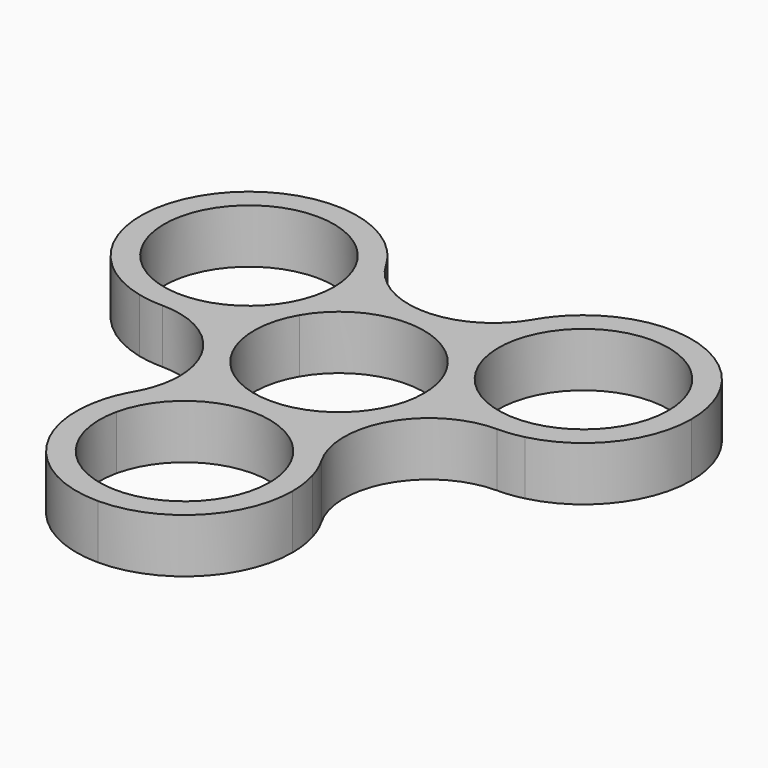
from build123d import *

# Parameters (mm, degrees)
F1_DEPTH = 7


# Not quite as in the source:
# - a feature names something its author has since deleted; it is built from what else it names


with BuildPart() as f1:
    # F0 (on Top) → F1 (new body)
    with BuildSketch(Plane.XY):
        with BuildLine():
            ThreePointArc((9.5262796516, 5.4999996362), (10.6251841435, 2.8470092933), (11, 0))
            ThreePointArc((11, 0), (7.7781745931, -7.7781745931), (0, -11))
            ThreePointArc((0, -11), (6.9999999972, -12.8756443454), (12.1243556497, -17.9999999943))
            ThreePointArc((12.1243556497, -17.9999999943), (12.1243556546, -6.9999999972), (21.6506350946, -1.5))
            ThreePointArc((21.6506350946, -1.5), (14.6506352765, 0.375644242), (9.5262796516, 5.4999996362))
        make_face()
        with BuildLine():
            ThreePointArc((-9.5262796375, 5.4999996607), (1.41e-08, 11), (9.5262796516, 5.4999996362))
            ThreePointArc((9.5262796516, 5.4999996362), (7.6506350946, 12.4999999615), (9.5262796131, 19.500000297))
            ThreePointArc((9.5262796131, 19.500000297), (-4.54e-08, 14), (-9.5262796585, 19.5000003756))
            ThreePointArc((-9.5262796585, 19.5000003756), (-8.1276735827, 16.1234668409), (-7.6506350946, 12.5))
            ThreePointArc((-7.6506350946, 12.5), (-8.1276735773, 8.8765331793), (-9.5262796375, 5.4999996607))
        make_face()
        with BuildLine():
            ThreePointArc((9.5262796131, 19.500000297), (7.6506350946, 12.4999999615), (9.5262796516, 5.4999996362))
            ThreePointArc((9.5262796516, 5.4999996362), (14.6506352765, 0.375644242), (21.6506350946, -1.5))
            ThreePointArc((21.6506350946, -1.5), (23.3252484864, -1.3994845224), (24.9758155118, -1.0993814269))
            ThreePointArc((24.9758155118, -1.0993814269), (24.9939531467, -0.5498237016), (25, 0))
            ThreePointArc((25, 0), (24.9800177424, 0.9993565887), (24.9201029127, 1.9971156254))
            ThreePointArc((24.9201029127, 1.9971156254), (12.124355653, 7), (14.1896043222, 20.5828843746))
            ThreePointArc((14.1896043222, 20.5828843746), (12.8874554167, 21.4222662872), (11.5358155118, 22.1793814269))
            ThreePointArc((11.5358155118, 22.1793814269), (10.4506351975, 20.9000001372), (9.5262796131, 19.500000297))
        make_face()
        with BuildLine():
            ThreePointArc((-12.1243556177, -17.999999939), (-6.9999999695, -12.8756443294), (0, -11))
            ThreePointArc((0, -11), (-9.5262793437, -5.5000001697), (-9.5262796375, 5.4999996607))
            ThreePointArc((-9.5262796375, 5.4999996607), (-14.6506352643, 0.3756442491), (-21.6506350946, -1.5))
            ThreePointArc((-21.6506350946, -1.5), (-13.8724605016, -4.7218254069), (-10.6506350946, -12.5))
            ThreePointArc((-10.6506350946, -12.5), (-11.0254509963, -15.3470094621), (-12.1243556177, -17.999999939))
        make_face()
        with BuildLine():
            ThreePointArc((12.1243556497, -17.9999999943), (6.9999999972, -12.8756443454), (0, -11))
            ThreePointArc((0, -11), (-6.9999999695, -12.8756443294), (-12.1243556177, -17.999999939))
            ThreePointArc((-12.1243556177, -17.999999939), (-12.8746133779, -19.5005154452), (-13.44, -21.08))
            ThreePointArc((-13.44, -21.08), (-12.108499103, -21.8719969247), (-10.7304985905, -22.58))
            ThreePointArc((-10.7304985905, -22.58), (0, -14), (10.7304985905, -22.58))
            ThreePointArc((10.7304985905, -22.58), (12.108499103, -21.8719969247), (13.44, -21.08))
            ThreePointArc((13.44, -21.08), (12.8746133905, -19.5005154746), (12.1243556497, -17.9999999943))
        make_face()
        with BuildLine():
            ThreePointArc((-21.6506350946, -1.5), (-14.6506352643, 0.3756442491), (-9.5262796375, 5.4999996607))
            ThreePointArc((-9.5262796375, 5.4999996607), (-8.1276735773, 8.8765331793), (-7.6506350946, 12.5))
            ThreePointArc((-7.6506350946, 12.5), (-8.1276735827, 16.1234668409), (-9.5262796585, 19.5000003756))
            ThreePointArc((-9.5262796585, 19.5000003756), (-10.4506352247, 20.9000001735), (-11.5358155118, 22.1793814269))
            ThreePointArc((-11.5358155118, 22.1793814269), (-12.8874554167, 21.4222662872), (-14.1896043222, 20.5828843746))
            ThreePointArc((-14.1896043222, 20.5828843746), (-11.5741441752, 16.9118398375), (-10.6506350946, 12.5))
            ThreePointArc((-10.6506350946, 12.5), (-15.1300578962, 3.6409891636), (-24.9201029127, 1.9971156254))
            ThreePointArc((-24.9201029127, 1.9971156254), (-24.9959545198, 0.4497306374), (-24.9758155118, -1.0993814269))
            ThreePointArc((-24.9758155118, -1.0993814269), (-23.3252484864, -1.3994845224), (-21.6506350946, -1.5))
        make_face()
        with BuildLine():
            ThreePointArc((33.7749911327, 19.499999333), (23.3252488687, 26.3994844763), (11.5358155118, 22.1793814269))
            ThreePointArc((11.5358155118, 22.1793814269), (12.8874554167, 21.4222662872), (14.1896043222, 20.5828843746))
            ThreePointArc((14.1896043222, 20.5828843746), (26.0624749321, 22.5764909194), (32.6506350946, 12.5))
            ThreePointArc((32.6506350946, 12.5), (30.509645931, 5.9794228016), (24.9201029127, 1.9971156254))
            ThreePointArc((24.9201029127, 1.9971156254), (24.9800177424, 0.9993565887), (25, 0))
            ThreePointArc((25, 0), (24.9939531467, -0.5498237016), (24.9758155118, -1.0993814269))
            ThreePointArc((24.9758155118, -1.0993814269), (32.6631853406, 3.8557107244), (35.6506350946, 12.5))
            ThreePointArc((35.6506350946, 12.5), (35.1735967623, 16.1234662595), (33.7749911327, 19.499999333))
        make_face()
        with BuildLine():
            ThreePointArc((14, -25), (13.8592929113, -23.0201010127), (13.44, -21.08))
            ThreePointArc((13.44, -21.08), (12.108499103, -21.8719969247), (10.7304985905, -22.58))
            ThreePointArc((10.7304985905, -22.58), (10.9324170359, -23.782519917), (11, -25))
            ThreePointArc((11, -25), (-1.217480083, -35.9324170359), (-10.7304985905, -22.58))
            ThreePointArc((-10.7304985905, -22.58), (-12.108499103, -21.8719969247), (-13.44, -21.08))
            ThreePointArc((-13.44, -21.08), (-11.2000000155, -33.3999999793), (-5.18e-08, -39))
            ThreePointArc((-5.18e-08, -39), (9.8994949183, -34.8994949549), (14, -25))
        make_face()
        with BuildLine():
            ThreePointArc((-33.7749911175, 19.4999993593), (-34.5252483411, 7.0005151375), (-24.9758155118, -1.0993814269))
            ThreePointArc((-24.9758155118, -1.0993814269), (-24.9959545198, 0.4497306374), (-24.9201029127, 1.9971156254))
            ThreePointArc((-24.9201029127, 1.9971156254), (-31.1769145362, 18), (-14.1896043222, 20.5828843746))
            ThreePointArc((-14.1896043222, 20.5828843746), (-12.8874554167, 21.4222662872), (-11.5358155118, 22.1793814269))
            ThreePointArc((-11.5358155118, 22.1793814269), (-23.3252488536, 26.3994844781), (-33.7749911175, 19.4999993593))
        make_face()
    extrude(amount=F1_DEPTH)


solid = f1.part
